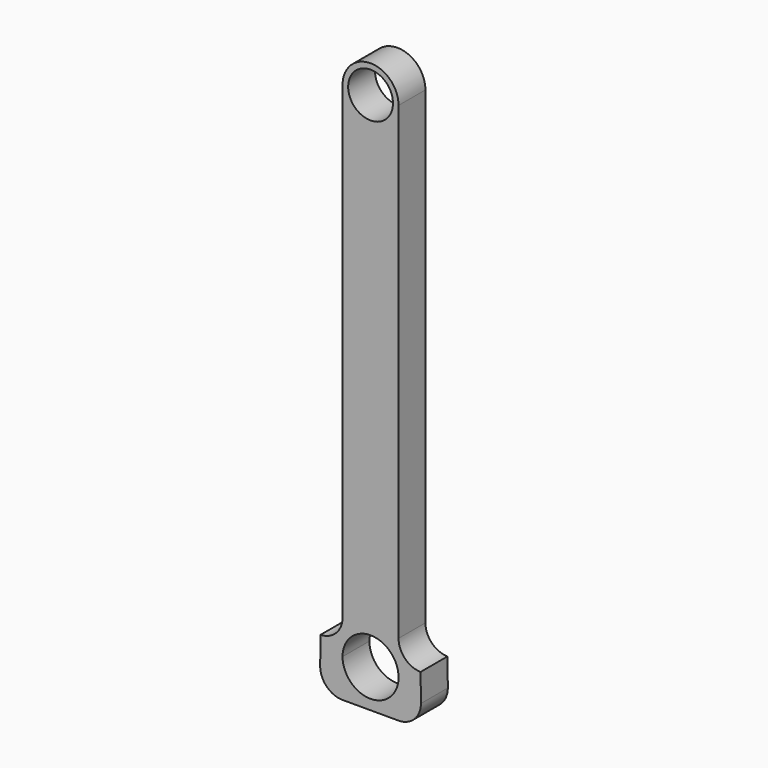
from build123d import *

# Parameters (mm, degrees)
F0_R     = 10
F1_DEPTH = 15


# Not quite as in the source:
# - a feature names something its author has since deleted; it is built from what else it names


with BuildPart() as f1:
    # F0 (on Front) → F1 (new body)
    with BuildSketch(Plane.XZ):
        with BuildLine():
            ThreePointArc((-12.4862537895, 224.2308067578), (0.2931105859, 212.3203037661), (12.5, 224.8168667409))
            ThreePointArc((12.5, 224.8168667409), (0.293876674, 237.3134117235), (-12.4861818401, 225.404457633))
            Line((-12.4861818401, 225.404457633), (-12.4862537895, 224.2308067578))
        make_face()
        with Locations((0, 224.8168667409)):
            Circle(F0_R, mode=Mode.SUBTRACT)
        with BuildLine():
            Line((12.5, 15.3332800892), (12.5, 224.8168667409))
            ThreePointArc((12.5, 224.8168667409), (0.2931105859, 212.3203037661), (-12.4862537895, 224.2308067578))
            Line((-12.4862537895, 224.2308067578), (-12.4990556694, 15.4044580276))
            ThreePointArc((-12.4990556694, 15.4044580276), (-15.36849483, 8.3940010786), (-22.3294631759, 5.4065092509))
            Line((-22.3294631759, 5.4065092509), (-22.5, -7))
            ThreePointArc((-22.5, -7), (-19.5710678119, -14.0710678119), (-12.5, -17))
            Line((-12.5, -17), (12.5, -17))
            ThreePointArc((12.5, -17), (19.5710678119, -14.0710678119), (22.5, -7))
            Line((22.5, -7), (22.3300547766, 5.3347242624))
            ThreePointArc((22.3300547766, 5.3347242624), (15.3691006095, 8.3225544574), (12.5, 15.3332800892))
        make_face()
        with BuildLine():
            ThreePointArc((-12.4999999765, 0.0007662994), (0.0003831497, 12.4999999941), (12.5, 0))
            ThreePointArc((12.5, 0), (0, -12.5), (-12.5, 0))
            Line((-12.5000000235, 0), (-12.4999999765, 0.0007662994))
        make_face(mode=Mode.SUBTRACT)
    extrude(amount=F1_DEPTH)


solid = f1.part
